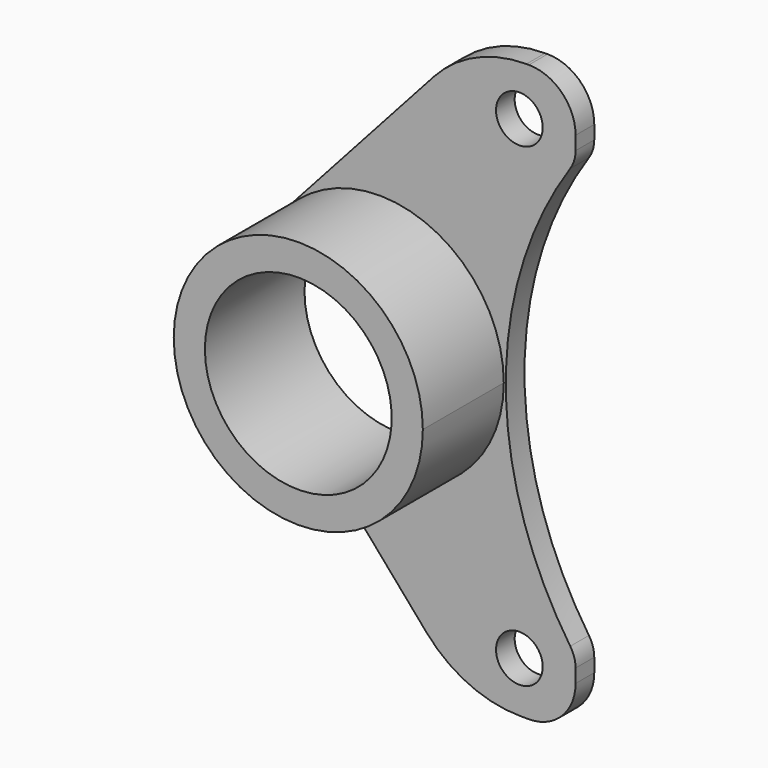
from build123d import *

# Parameters (mm, degrees)
F0_R     = 1.5
F1_DEPTH = 1.5
F2_DEPTH = 8
F3_R     = 8
F4_R     = 3
F5_R     = 2
F6_R     = 8
F7_R     = 3
F8_R     = 2


with BuildPart() as f1:
    # F0 (on Front) → F1 (new body)
    with BuildSketch(Plane.XZ):
        with BuildLine():
            Line((-26.0642077774, -18.5), (-18.8888516277, -18.5))
            Line((-18.8888516277, -18.5), (-18.8888516277, -14))
            ThreePointArc((-18.8888516277, -14), (-23.3701047123, 0), (-18.8888516277, 14))
            Line((-18.8888516277, 14), (-18.8888516277, 18.5))
            Line((-18.8888516277, 18.5), (-25.6080199033, 18.5))
            Line((-25.6080199033, 18.5), (-37.3901407018, 5.4135240382))
            ThreePointArc((-37.3901407018, 5.4135240382), (-28.5949290555, 7.4538958141), (-23.5, 0))
            ThreePointArc((-23.5, 0), (-28.6715728753, -7.4833147735), (-37.5, -5.2915026221))
            Line((-37.5, -5.2915026221), (-37.5, -5.2920114501))
            Line((-37.5, -5.2920114501), (-26.0642077774, -18.5))
        make_face()
        with Locations((-22.5, -15.25)):
            Circle(F0_R, mode=Mode.SUBTRACT)
        with Locations((-22.5, 15.25)):
            Circle(F0_R, mode=Mode.SUBTRACT)
    extrude(amount=F1_DEPTH)

    # F0 (on Front) → F2 (join)
    with BuildSketch(Plane.XZ):
        with BuildLine():
            Line((-37.5, 0), (-37.5, -5.2915026221))
            ThreePointArc((-37.5, -5.2915026221), (-28.6715728753, -7.4833147735), (-23.5, 0))
            ThreePointArc((-23.5, 0), (-28.5949290555, 7.4538958141), (-37.3901407018, 5.4135240382))
            Line((-37.3901407018, 5.4135240382), (-37.5, 5.2915026221))
            Line((-37.5, 5.2915026221), (-37.5, 0))
        make_face()
        with BuildLine():
            ThreePointArc((-25.5, 0), (-31.5, -6), (-37.5, 0))
            ThreePointArc((-37.5, 0), (-31.5, 6), (-25.5, 0))
        make_face(mode=Mode.SUBTRACT)
        with BuildLine():
            ThreePointArc((-37.5, 5.2915026221), (-39.5, 0), (-37.5, -5.2915026221))
            Line((-37.5, -5.2915026221), (-37.5, 0))
            Line((-37.5, 0), (-37.5, 5.2915026221))
        make_face()
    extrude(amount=F2_DEPTH)

    # F3
    f3_edges = [f1.edges().sort_by_distance(p)[0] for p in [
        (-26.064208, -0.75, -18.5),
    ]]
    fillet(f3_edges, radius=F3_R)

    # F4
    f4_edges = [f1.edges().sort_by_distance(p)[0] for p in [
        (-18.888852, -0.75, -18.5),
    ]]
    fillet(f4_edges, radius=F4_R)

    # F5
    f5_edges = [f1.edges().sort_by_distance(p)[0] for p in [
        (-18.888852, -0.75, 14),
    ]]
    fillet(f5_edges, radius=F5_R)

    # F6
    f6_edges = [f1.edges().sort_by_distance(p)[0] for p in [
        (-25.60802, -0.75, 18.5),
    ]]
    fillet(f6_edges, radius=F6_R)

    # F7
    f7_edges = [f1.edges().sort_by_distance(p)[0] for p in [
        (-18.888852, -0.75, 18.5),
    ]]
    fillet(f7_edges, radius=F7_R)

    # F8
    f8_edges = [f1.edges().sort_by_distance(p)[0] for p in [
        (-18.888852, -0.75, -14),
    ]]
    fillet(f8_edges, radius=F8_R)


solid = f1.part
